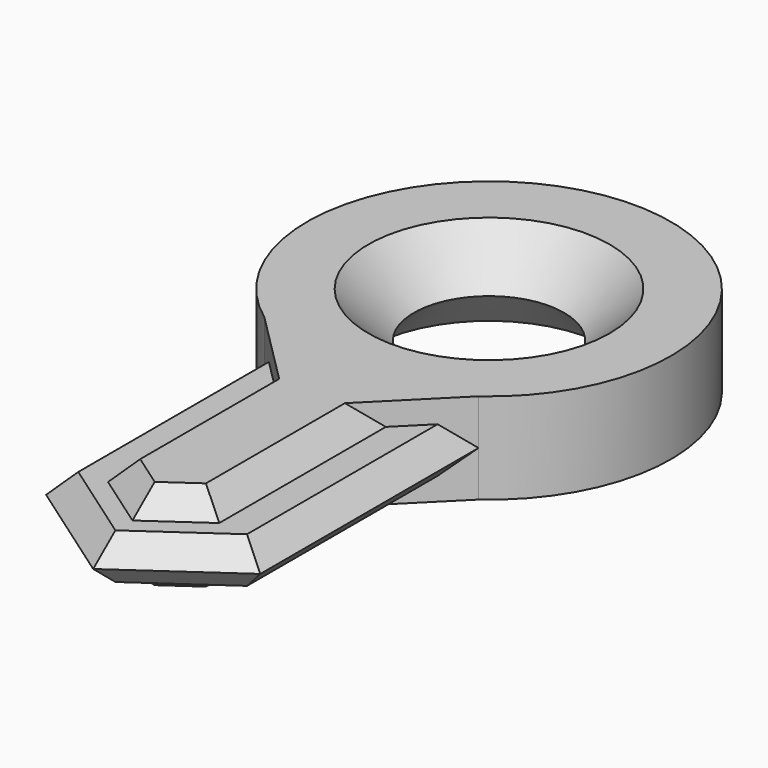
from build123d import *

# Parameters (mm, degrees)
F0_R     = 4.1965730186
F1_DEPTH = 2.54
F2_DEPTH = 1.27
F3_SIZE  = 1.26999
F4_SIZE  = 2.53999


# Not quite as in the source:
# - a fillet or chamfer is up to 0.001 mm smaller than in the source, because OpenCascade refuses the exact size


with BuildPart() as f1:
    # F0 (on Top) → F1 (new body, symmetric)
    with BuildSketch(Plane.XY):
        with BuildLine():
            ThreePointArc((0, 49.7234201631), (-9.6606227132, 42.7095239111), (-5.9829372688, 31.3518392168))
            Line((-5.9829372688, 31.3518392168), (-1.8358110683, 27.2047130163))
            Line((-1.8358110683, 27.2047130163), (-1.8358110683, 17.501438998))
            Line((-1.8358110683, 17.501438998), (0, 16.2159902493))
            Line((0, 16.2159902493), (1.8358110683, 17.501438998))
            Line((1.8358110683, 17.501438998), (1.8358110683, 27.2047130163))
            Line((1.8358110683, 27.2047130163), (5.9829372688, 31.3518392168))
            ThreePointArc((5.9829372688, 31.3518392168), (9.6606227132, 42.7095239111), (0, 49.7234201631))
        make_face()
        with Locations((0, 39.5634201631)):
            Circle(F0_R, mode=Mode.SUBTRACT)
    extrude(amount=F1_DEPTH, both=True)

    # F0 (on Top) → F2 (join, symmetric)
    with BuildSketch(Plane.XY):
        Polygon((-1.8358110683, 27.2047130163), (-5.9829372688, 31.3518392168), (-5.9829372688, 16.1118392168), (0, 11.9225414406), (5.9829372688, 16.1118392168), (5.9829372688, 31.3518392168), (1.8358110683, 27.2047130163), (1.8358110683, 17.501438998), (0, 16.2159902493), (-1.8358110683, 17.501438998), align=None)
    extrude(amount=F2_DEPTH, both=True)

    # F3 (size 1.27 in the source; OpenCascade refuses exactly that, so slightly less here)
    f3_edges = [f1.edges().sort_by_distance(p)[0] for p in [
        (0.917906, 16.858715, 1.27),
        (-0.917906, 16.858715, 1.27),
        (1.835811, 22.353076, 1.27),
        (-1.835811, 22.353076, 1.27),
        (5.982937, 23.731839, 1.27),
        (-5.982937, 23.731839, 1.27),
        (-2.991469, 14.01719, 1.27),
        (2.991469, 14.01719, 1.27),
        (2.991469, 14.01719, -1.27),
        (5.982937, 23.731839, -1.27),
        (0.917906, 16.858715, -1.27),
        (1.835811, 22.353076, -1.27),
        (-0.917906, 16.858715, -1.27),
        (-1.835811, 22.353076, -1.27),
        (-5.982937, 23.731839, -1.27),
        (-2.991469, 14.01719, -1.27),
    ]]
    chamfer(f3_edges, length=F3_SIZE)

    # F4 (size 2.54 in the source; OpenCascade refuses exactly that, so slightly less here)
    f4_edges = [f1.edges().sort_by_distance(p)[0] for p in [
        (-4.196573, 39.56342, 2.54),
        (-4.196573, 39.56342, -2.54),
    ]]
    chamfer(f4_edges, length=F4_SIZE)


solid = f1.part
